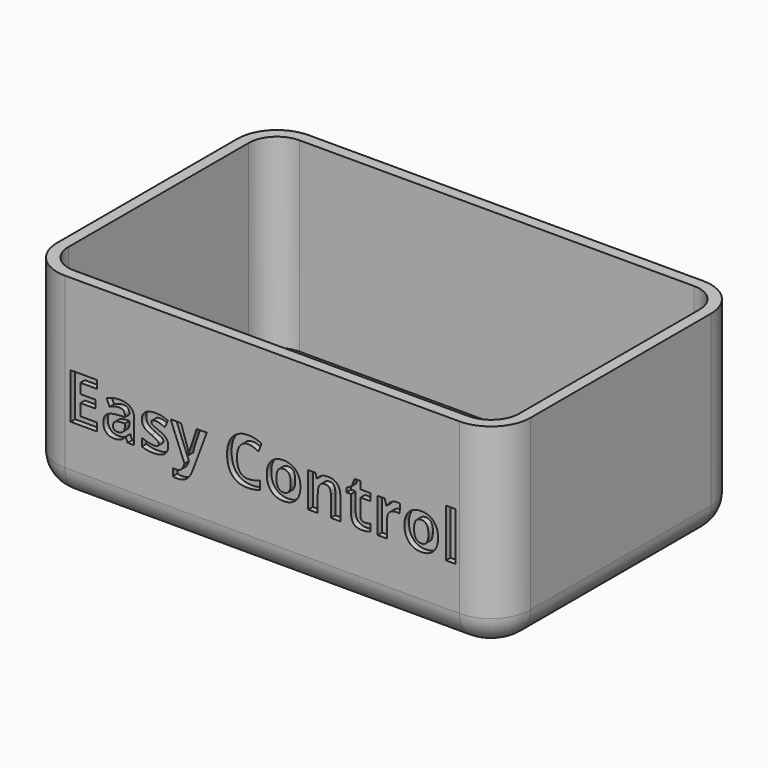
from build123d import *

# Parameters (mm, degrees)
F1_DEPTH     = 4
F2_DEPTH     = 70
F3_TEXT_SIZE = 22.5709751367
F4_DEPTH     = 2
F5_R         = 10


# Not quite as in the source:
# - Text() gives the source's letters only with a copy of the font that has no kerning and outlines rounded to 1/6400 em; it was checked with that copy


with BuildPart() as f1:
    # F0 (on Top) → F1 (new body)
    with BuildSketch(Plane.XY):
        with BuildLine():
            ThreePointArc((80, 40), (77.0710678119, 47.0710678119), (70, 50))
            Line((70, 50), (-70, 50))
            ThreePointArc((-70, 50), (-77.0710678119, 47.0710678119), (-80, 40))
            Line((-80, 40), (-80, -40))
            ThreePointArc((-80, -40), (-77.0710678119, -47.0710678119), (-70, -50))
            Line((-70, -50), (70, -50))
            ThreePointArc((70, -50), (77.0710678119, -47.0710678119), (80, -40))
            Line((80, -40), (80, 40))
        make_face()
    extrude(amount=F1_DEPTH)

    # F0 (on Top) → F2 (join)
    with BuildSketch(Plane.XY):
        with BuildLine():
            Line((84, -40), (84, 40))
            ThreePointArc((84, 40), (79.8994949366, 49.8994949366), (70, 54))
            Line((70, 54), (-70, 54))
            ThreePointArc((-70, 54), (-79.8994949366, 49.8994949366), (-84, 40))
            Line((-84, 40), (-84, -40))
            ThreePointArc((-84, -40), (-79.8994949366, -49.8994949366), (-70, -54))
            Line((-70, -54), (70, -54))
            ThreePointArc((70, -54), (79.8994949366, -49.8994949366), (84, -40))
        make_face()
        with BuildLine():
            Line((-70, 50), (70, 50))
            ThreePointArc((70, 50), (77.0710678119, 47.0710678119), (80, 40))
            Line((80, 40), (80, -40))
            ThreePointArc((80, -40), (77.0710678119, -47.0710678119), (70, -50))
            Line((70, -50), (-70, -50))
            ThreePointArc((-70, -50), (-77.0710678119, -47.0710678119), (-80, -40))
            Line((-80, -40), (-80, 40))
            ThreePointArc((-80, 40), (-77.0710678119, 47.0710678119), (-70, 50))
        make_face(mode=Mode.SUBTRACT)
    extrude(amount=F2_DEPTH)

    # F3 (on face) → F4 (cut)
    with BuildSketch(Plane.XZ.offset(54)):
        with Locations((-70, 25)):
            Text('Easy Control', F3_TEXT_SIZE, font='Open Sans', font_style=FontStyle.BOLD, text_align=(TextAlign.LEFT, TextAlign.BOTTOM))
    extrude(amount=-F4_DEPTH, mode=Mode.SUBTRACT)

    # F5
    f5_edges = [f1.edges().sort_by_distance(p)[0] for p in [
        (0, -54, 0),
    ]]
    fillet(f5_edges, radius=F5_R)


solid = f1.part
